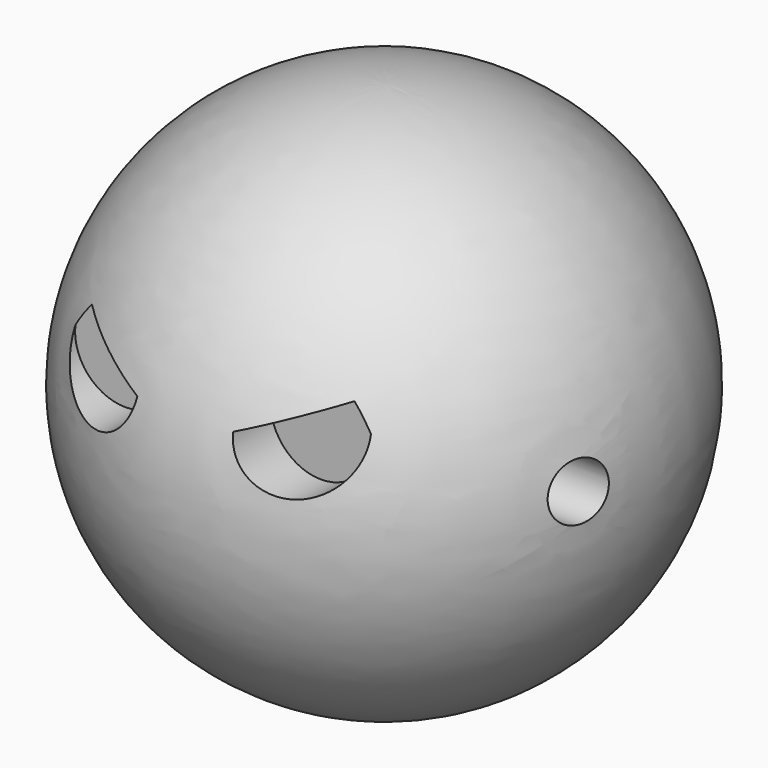
from build123d import *

# Parameters (mm, degrees)
F5_DEPTH  = 13.97
F6_R      = 1.6
F7_DEPTH  = 15.24
F8_W      = 36.1250601709
F8_H      = 9.7824148252
F9_DEPTH  = 76.2
F10_R     = 1.5
F11_DEPTH = 2.794


# Not quite as in the source:
# - ends of sketch curves that miss each other by under 0.0002 mm in the source are joined


with BuildPart() as f1:
    # F0 (on Front) → F1 (revolve)
    with BuildSketch(Plane.XZ):
        with BuildLine():
            Line((0, 30), (0, 0))
            ThreePointArc((0, 0), (15.0000006192, 15), (0, 30))
        make_face()
    revolve(axis=Axis((0, 0, 15), (0, 0, 1)))

    # F4 (on offset) → F5 (cut)
    with BuildSketch(Plane.XZ.offset(25.4)):
        with BuildLine():
            ThreePointArc((-7.7757835388, 21.3449876755), (-6.6607308484, 16.8981042804), (-2.7180244215, 19.2375872284))
            Line((-2.7180244215, 19.2375872284), (-7.7757835388, 21.3449876755))
        make_face()
        with BuildLine():
            Line((7.7757835388, 21.3449876755), (2.7180244215, 19.2375872284))
            ThreePointArc((2.7180244215, 19.2375872284), (6.6607308484, 16.8981042804), (7.7757835388, 21.3449876755))
        make_face()
    extrude(amount=-F5_DEPTH, mode=Mode.SUBTRACT)

    # F6 (on offset) → F7 (cut)
    with BuildSketch(Plane.YZ.offset(25.4)):
        with Locations((-4.0855947882, 15.938160941)):
            Circle(F6_R)
    extrude(amount=-F7_DEPTH, mode=Mode.SUBTRACT)

    # F8 (on offset) → F9 (cut)
    with BuildSketch(Plane.XZ.offset(25.4)):
        with Locations((1.2260917574, -4.0021650784)):
            Rectangle(F8_W, F8_H)
    extrude(amount=-F9_DEPTH, mode=Mode.SUBTRACT)

    # F10 (on face) → F11 (cut)
    with BuildSketch(Plane(origin=(0, 0, 0.8890423342), x_dir=(1, 0, 0), z_dir=(0, 0, -1))):
        Circle(F10_R)
    extrude(amount=-F11_DEPTH, mode=Mode.SUBTRACT)


solid = f1.part
